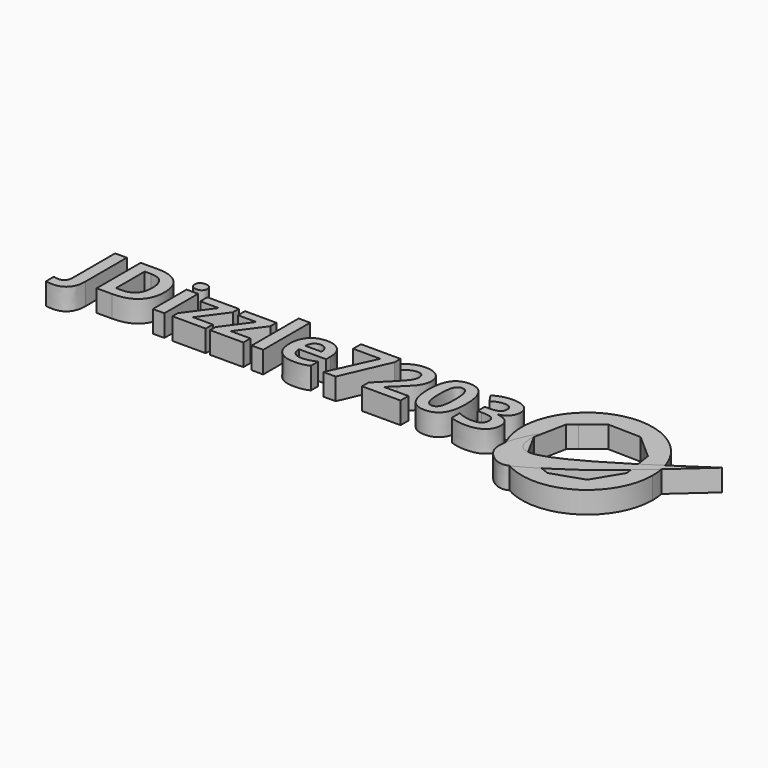
from build123d import *

# Parameters (mm, degrees)
F0_TEXT_SIZE = 90.1761852826
F1_DEPTH     = 25.4
F3_DEPTH     = 25.4


# Not quite as in the source:
# - Text() gives the source's letters only with a copy of the font that has no kerning and outlines rounded to 1/6400 em; it was checked with that copy


with BuildPart() as f1:
    # F0 (on Top) → F1 (new body)
    with BuildSketch(Plane.XY):
        with BuildLine():
            ThreePointArc((56.2546237322, -51.847082156), (71.2613069958, -27.8303565302), (76.5029582392, 0))
            ThreePointArc((76.5029582392, 0), (69.1386951738, 32.7497091439), (48.4636909037, 59.1943686793))
            Line((48.4636909037, 59.1943686793), (33.4886223529, 40.9035676225))
            Line((33.4886223529, 40.9035676225), (49.3216839982, 26.9869144113))
            Line((49.3216839982, 26.9869144113), (55.1294561593, -11.0301915412))
            Line((55.1294561593, -11.0301915412), (39.6233994926, -36.5189119134))
            Line((39.6233994926, -36.5189119134), (56.2546237322, -51.847082156))
        make_face()
        with BuildLine():
            Line((33.4886223529, 40.9035676225), (48.4636909037, 59.1943686793))
            ThreePointArc((48.4636909037, 59.1943686793), (-5.3564435794, 76.3152090447), (-56.2573097926, 51.8441676011))
            Line((-56.2573097926, 51.8441676011), (-39.2974084512, 36.214697033))
            Line((-39.2974084512, 36.214697033), (-18.0123019964, 53.2586053014))
            Line((-18.0123019964, 53.2586053014), (20.4357477448, 52.3765431846))
            Line((20.4357477448, 52.3765431846), (33.4886223529, 40.9035676225))
        make_face()
        with BuildLine():
            ThreePointArc((-54.7838240429, -53.3988318467), (1.0690157656, -76.4954889169), (56.2546237322, -51.847082156))
            Line((56.2546237322, -51.847082156), (39.6233994926, -36.5189119134))
            Line((39.6233994926, -36.5189119134), (35.1415430878, -43.8861482846))
            Line((35.1415430878, -43.8861482846), (-1.2894885492, -56.2072885055))
            Line((-1.2894885492, -56.2072885055), (-37.1171541629, -42.2284137602))
            Line((-37.1171541629, -42.2284137602), (-39.2759334149, -38.2829968642))
            Line((-39.2759334149, -38.2829968642), (-54.7838240429, -53.3988318467))
        make_face()
        with BuildLine():
            Line((-39.2974084512, 36.214697033), (-56.2573097926, 51.8441676011))
            ThreePointArc((-56.2573097926, 51.8441676011), (-76.4954611991, -1.0709973356), (-54.7838240429, -53.3988318467))
            Line((-54.7838240429, -53.3988318467), (-39.2759334149, -38.2829968642))
            Line((-39.2759334149, -38.2829968642), (-55.5772908327, -8.4903948999))
            Line((-55.5772908327, -8.4903948999), (-48.032195449, 29.2203740942))
            Line((-48.032195449, 29.2203740942), (-39.2974084512, 36.214697033))
        make_face()
        with Locations((-588.53495121, -28.1275678426)):
            Text('JDizzle7203', F0_TEXT_SIZE, font='Open Sans', font_style=FontStyle.BOLD, text_align=(TextAlign.LEFT, TextAlign.BOTTOM))
    extrude(amount=F1_DEPTH)


with BuildPart() as f3:
    # F2 (on Top) → F3 (new body)
    with BuildSketch(Plane.XY):
        with BuildLine():
            add(Edge.make_bspline(
                [(-55.5104166269, 0), (-56.0234726165, -9.4797036888), (-56.9711506082, -26.9898911483), (-31.0809468215, -47.2180686371), (52.8604842467, 8.959166936), (116.2481531501, 51.3809360564)],
                knots=[0, 0, 0, 0, 0.2242329142, 0.41418598, 1, 1, 1, 1], degree=3))
            add(Edge.make_bspline(
                [(-55.5104166269, 0), (-57.3444722284, -3.1159034796), (-61.6082439455, -10.3596866665), (-69.6959426013, -29.1609053546), (-71.5872713431, -53.5568203469), (-49.176653534, -70.9204372267), (-32.9844163808, -65.6386752168), (-4.9584978873, -48.2824723883), (19.8656772885, -31.807712816), (52.0279326797, -6.5164985597), (92.1642456295, 29.6682036684), (116.2481531501, 51.3809360564)],
                knots=[0, 0, 0, 0, 0.0704435923, 0.1637656984, 0.2631172064, 0.3639787591, 0.4454340684, 0.5630075235, 0.6757889209, 0.8054562297, 1, 1, 1, 1], degree=3))
        make_face()
    extrude(amount=F3_DEPTH)


solid = Compound([f1.part, f3.part])
